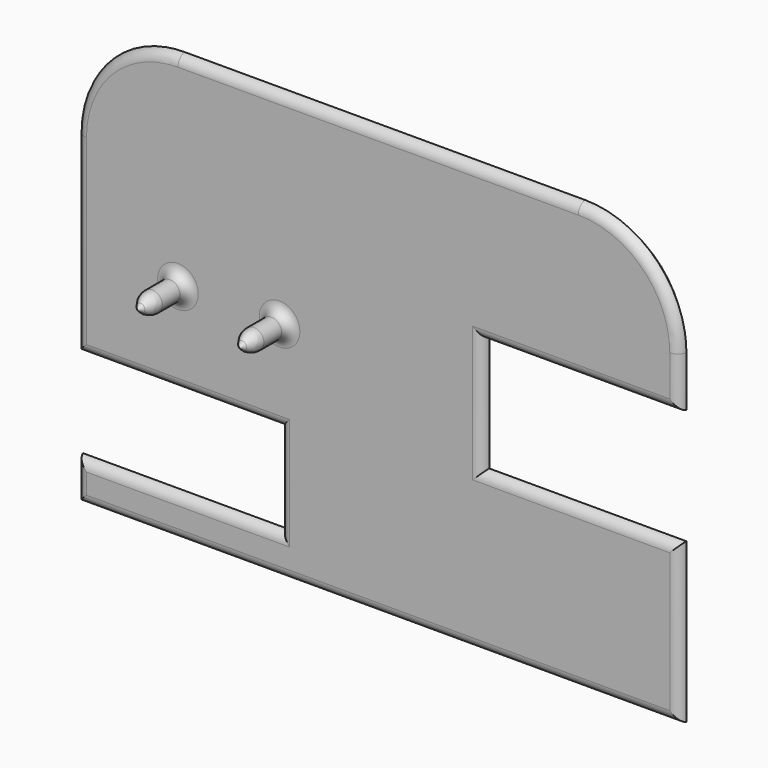
from build123d import *

# Parameters (mm, degrees)
F1_DEPTH      = 9
F2_R          = 5
F3_DEPTH      = 25
F4_W          = 103.9993347282
F4_H          = 56.6140824735
F5_DEPTH      = 25
F6_W          = 113.1558813547
F6_H          = 45.2373955332
F7_DEPTH      = 25
F8_R          = 5
F9_SIZE       = 5
F10_R         = 10
F11_T1_DEPTH  = 37.8584149398
F11_T3_DEPTH  = 109.8584149398
F11_T5_DEPTH  = 56.6140824735
F11_T7_DEPTH  = 104.1027474062
F11_T9_DEPTH  = 322.7168298797
F11_T11_DEPTH = 45.7168298797
F11_T13_DEPTH = 112.8584149398
F11_T15_DEPTH = 45.2373955332
F11_T17_DEPTH = 107.6210194067
F11_T19_DEPTH = 197
F11_T22_ANGLE = 90
F11_T24_ANGLE = 90
F11_T29_DEPTH = 122.7168298797
F11_T33_DEPTH = 69.4724974133
F11_T40_DEPTH = 69.4724974133
F11_T44_DEPTH = 122.7168298797
F11_T51_DEPTH = 58.095810473
F11_T55_DEPTH = 125.7168298797
F11_T62_DEPTH = 125.7168298797
F11_T66_DEPTH = 58.095810473


# Not quite as in the source:
# - a fillet or chamfer that OpenCascade refuses, or shapes differently, is made with other operations: its cross-section is extruded or revolved along the edge and cut away or added


with BuildPart() as f1:
    # F0 (on Front) → F1 (new body)
    with BuildSketch(Plane.XZ):
        with BuildLine():
            Line((100.0664040952, 56.5429037459), (-96.9335959048, 56.5429037459))
            ThreePointArc((-96.9335959048, 56.5429037459), (-132.2889349642, 41.8982428052), (-146.9335959048, 6.5429037459))
            Line((-146.9335959048, 6.5429037459), (-146.9335959048, -153.4570962541))
            Line((-146.9335959048, -153.4570962541), (150.0664040952, -153.4570962541))
            Line((150.0664040952, -153.4570962541), (150.0664040952, 6.5429037459))
            ThreePointArc((150.0664040952, 6.5429037459), (135.4217431545, 41.8982428052), (100.0664040952, 56.5429037459))
        make_face()
    extrude(amount=F1_DEPTH)

    # F2 (on face) → F3 (join)
    with BuildSketch(Plane.XZ.offset(9)):
        with Locations((-46.9335959048, -43.4570962541)):
            Circle(F2_R)
        with Locations((-96.9335959048, -43.4570962541)):
            Circle(F2_R)
    extrude(amount=F3_DEPTH)

    # F4 (on face) → F5 (cut)
    with BuildSketch(Plane.XZ.offset(9)):
        with Locations((105.0660714593, -46.7641374908)):
            Rectangle(F4_W, F4_H)
    extrude(amount=-F5_DEPTH, mode=Mode.SUBTRACT)

    # F6 (on face) → F7 (cut)
    with BuildSketch(Plane.XZ.offset(9)):
        with Locations((-103.5115365822, -110.8383984875)):
            Rectangle(F6_W, F6_H)
    extrude(amount=-F7_DEPTH, mode=Mode.SUBTRACT)

    # F8
    f8_edges = [f1.edges().sort_by_distance(p)[0] for p in [
        (150.066404, -9, -5.957096),
        (101.566404, -9, -18.457096),
        (53.066404, -9, -46.764137),
        (101.566404, -9, -75.071179),
        (150.066404, -9, -114.264137),
        (1.566404, -9, -153.457096),
        (-146.933596, -9, -143.457096),
        (-96.933596, -9, -133.457096),
        (-46.933596, -9, -110.838398),
        (-96.933596, -9, -88.219701),
        (-146.933596, -9, -40.838398),
        (-132.288935, -9, 41.898243),
        (1.566404, -9, 56.542904),
        (135.421743, -9, 41.898243),
        (-101.933596, -9, -43.457096),
        (-51.933596, -9, -43.457096),
    ]]
    fillet(f8_edges, radius=F8_R)

    # F9
    f9_edges = [f1.edges().sort_by_distance(p)[0] for p in [
        (-101.933596, -34, -43.457096),
        (-51.933596, -34, -43.457096),
    ]]
    chamfer(f9_edges, length=F9_SIZE)

    # F10
    f10_edges = [f1.edges().sort_by_distance(p)[0] for p in [
        (-94.433596, -31.5, -43.457096),
        (-101.933596, -29, -43.457096),
        (-44.433596, -31.5, -43.457096),
        (-51.933596, -29, -43.457096),
    ]]
    fillet(f10_edges, radius=F10_R)

    # F11: chamfer of 5 on 14 edges, made by hand

    # F11_s2 → F11_t1 (cut)
    with BuildSketch(Plane.XY.offset(-31.3155111939)):
        Polygon((150.0664040952, -5), (145.0664040952, 0), (150.0664040952, 0), align=None)
    extrude(amount=F11_T1_DEPTH, mode=Mode.SUBTRACT)

    # F11_s4 → F11_t3 (cut)
    with BuildSketch(Plane.YZ.offset(53.0664040952)):
        Polygon((-5, -18.4570962541), (0, -13.4570962541), (0, -18.4570962541), align=None)
        Polygon((-5, -75.0711787276), (0, -80.0711787276), (0, -75.0711787276), align=None)
    extrude(amount=F11_T3_DEPTH, mode=Mode.SUBTRACT)

    # F11_s6 → F11_t5 (cut)
    with BuildSketch(Plane.XY.offset(-75.0711787276)):
        Polygon((53.0664040952, -5), (48.0664040952, 0), (53.0664040952, 0), align=None)
    extrude(amount=F11_T5_DEPTH, mode=Mode.SUBTRACT)

    # F11_s8 → F11_t7 (cut)
    with BuildSketch(Plane.XY.offset(-166.3155111939)):
        Polygon((150.0664040952, -5), (145.0664040952, 0), (150.0664040952, 0), align=None)
    extrude(amount=F11_T7_DEPTH, mode=Mode.SUBTRACT)

    # F11_s10 → F11_t9 (cut)
    with BuildSketch(Plane.YZ.offset(-159.7920108447)):
        Polygon((-5, -153.4570962541), (0, -148.4570962541), (0, -153.4570962541), align=None)
    extrude(amount=F11_T9_DEPTH, mode=Mode.SUBTRACT)

    # F11_s12 → F11_t11 (cut)
    with BuildSketch(Plane.XY.offset(-166.3155111939)):
        Polygon((-146.9335959048, -5), (-141.9335959048, 0), (-146.9335959048, 0), align=None)
    extrude(amount=F11_T11_DEPTH, mode=Mode.SUBTRACT)

    # F11_s14 → F11_t13 (cut)
    with BuildSketch(Plane.YZ.offset(-159.7920108447)):
        Polygon((-5, -133.4570962541), (0, -138.4570962541), (0, -133.4570962541), align=None)
        Polygon((-5, -88.2197007209), (0, -83.2197007209), (0, -88.2197007209), align=None)
    extrude(amount=F11_T13_DEPTH, mode=Mode.SUBTRACT)

    # F11_s16 → F11_t15 (cut)
    with BuildSketch(Plane.XY.offset(-133.4570962541)):
        Polygon((-46.9335959048, -5), (-41.9335959048, 0), (-46.9335959048, 0), align=None)
    extrude(amount=F11_T15_DEPTH, mode=Mode.SUBTRACT)

    # F11_s18 → F11_t17 (cut)
    with BuildSketch(Plane.XY.offset(-101.0781156608)):
        Polygon((-146.9335959048, -5), (-141.9335959048, 0), (-146.9335959048, 0), align=None)
    extrude(amount=F11_T17_DEPTH, mode=Mode.SUBTRACT)

    # F11_s20 → F11_t19 (cut)
    with BuildSketch(Plane.YZ.offset(-96.9335959048)):
        Polygon((-5, 56.5429037459), (0, 51.5429037459), (0, 56.5429037459), align=None)
    extrude(amount=F11_T19_DEPTH, mode=Mode.SUBTRACT)

    # F11_s21 → F11_t22 (revolve, cut)
    with BuildSketch(Plane.YZ.offset(-96.9335959048)):
        Polygon((-5, 56.5429037459), (0, 51.5429037459), (0, 56.5429037459), align=None)
    revolve(axis=Axis((-96.9335959048, 0, 6.5429037459), (0, -1, 0)), revolution_arc=F11_T22_ANGLE, mode=Mode.SUBTRACT)

    # F11_s23 → F11_t24 (revolve, cut)
    with BuildSketch(Plane.XY.offset(6.5429037459)):
        Polygon((150.0664040952, -5), (145.0664040952, 0), (150.0664040952, 0), align=None)
    revolve(axis=Axis((100.0664040952, 0, 6.5429037459), (0, -1, 0)), revolution_arc=F11_T24_ANGLE, mode=Mode.SUBTRACT)


with BuildPart() as f11_tool27:
    # F11_s28 → F11_t29 (new body)
    with BuildSketch(Plane.YZ.offset(162.924819035)):
        Polygon((-5, -18.4570962541), (0, -13.4570962541), (0, -18.4570962541), align=None)
    extrude(amount=-F11_T29_DEPTH)

    split(bisect_by=Plane.YZ.offset(53.0664040952), keep=Keep.BOTTOM)


with BuildPart() as f11_tool31:
    # F11_s32 → F11_t33 (new body)
    with BuildSketch(Plane.XY.offset(-5.5986813143)):
        Polygon((53.0664040952, -5), (48.0664040952, 0), (53.0664040952, 0), align=None)
    extrude(amount=-F11_T33_DEPTH)

    split(bisect_by=Plane.XY.offset(-18.4570962541), keep=Keep.TOP)


with BuildPart() as f11_tool27_1:
    add(f11_tool27.part)

    # F11_t35: intersect F11_tool31
    add(f11_tool31.part, mode=Mode.INTERSECT)


with BuildPart() as f1_1:
    add(f1.part)

    # F11_t25: cut F11_tool27
    add(f11_tool27_1.part, mode=Mode.SUBTRACT)


with BuildPart() as f11_tool38:
    # F11_s39 → F11_t40 (new body)
    with BuildSketch(Plane.XY.offset(-18.4570962541)):
        Polygon((53.0664040952, -5), (48.0664040952, 0), (53.0664040952, 0), align=None)
    extrude(amount=-F11_T40_DEPTH)

    split(bisect_by=Plane.XY.offset(-75.0711787276), keep=Keep.BOTTOM)


with BuildPart() as f11_tool42:
    # F11_s43 → F11_t44 (new body)
    with BuildSketch(Plane.YZ.offset(40.2079891553)):
        Polygon((-5, -75.0711787276), (0, -80.0711787276), (0, -75.0711787276), align=None)
    extrude(amount=F11_T44_DEPTH)

    split(bisect_by=Plane.YZ.offset(53.0664040952), keep=Keep.BOTTOM)


with BuildPart() as f11_tool38_1:
    add(f11_tool38.part)

    # F11_t46: intersect F11_tool42
    add(f11_tool42.part, mode=Mode.INTERSECT)


with BuildPart() as f1_2:
    add(f1_1.part)

    # F11_t36: cut F11_tool38
    add(f11_tool38_1.part, mode=Mode.SUBTRACT)


with BuildPart() as f11_tool49:
    # F11_s50 → F11_t51 (new body)
    with BuildSketch(Plane.XY.offset(-146.3155111939)):
        Polygon((-46.9335959048, -5), (-41.9335959048, 0), (-46.9335959048, 0), align=None)
    extrude(amount=F11_T51_DEPTH)

    split(bisect_by=Plane.XY.offset(-133.4570962541), keep=Keep.BOTTOM)


with BuildPart() as f11_tool53:
    # F11_s54 → F11_t55 (new body)
    with BuildSketch(Plane.YZ.offset(-159.7920108447)):
        Polygon((-5, -133.4570962541), (0, -138.4570962541), (0, -133.4570962541), align=None)
    extrude(amount=F11_T55_DEPTH)

    split(bisect_by=Plane.YZ.offset(-46.9335959048), keep=Keep.TOP)


with BuildPart() as f11_tool49_1:
    add(f11_tool49.part)

    # F11_t57: intersect F11_tool53
    add(f11_tool53.part, mode=Mode.INTERSECT)


with BuildPart() as f1_3:
    add(f1_2.part)

    # F11_t47: cut F11_tool49
    add(f11_tool49_1.part, mode=Mode.SUBTRACT)


with BuildPart() as f11_tool60:
    # F11_s61 → F11_t62 (new body)
    with BuildSketch(Plane.YZ.offset(-34.075180965)):
        Polygon((-5, -88.2197007209), (0, -83.2197007209), (0, -88.2197007209), align=None)
    extrude(amount=-F11_T62_DEPTH)

    split(bisect_by=Plane.YZ.offset(-46.9335959048), keep=Keep.TOP)


with BuildPart() as f11_tool64:
    # F11_s65 → F11_t66 (new body)
    with BuildSketch(Plane.XY.offset(-133.4570962541)):
        Polygon((-46.9335959048, -5), (-41.9335959048, 0), (-46.9335959048, 0), align=None)
    extrude(amount=F11_T66_DEPTH)

    split(bisect_by=Plane.XY.offset(-88.2197007209), keep=Keep.TOP)


with BuildPart() as f11_tool60_1:
    add(f11_tool60.part)

    # F11_t68: intersect F11_tool64
    add(f11_tool64.part, mode=Mode.INTERSECT)


with BuildPart() as f1_4:
    add(f1_3.part)

    # F11_t58: cut F11_tool60
    add(f11_tool60_1.part, mode=Mode.SUBTRACT)


solid = f1_4.part
